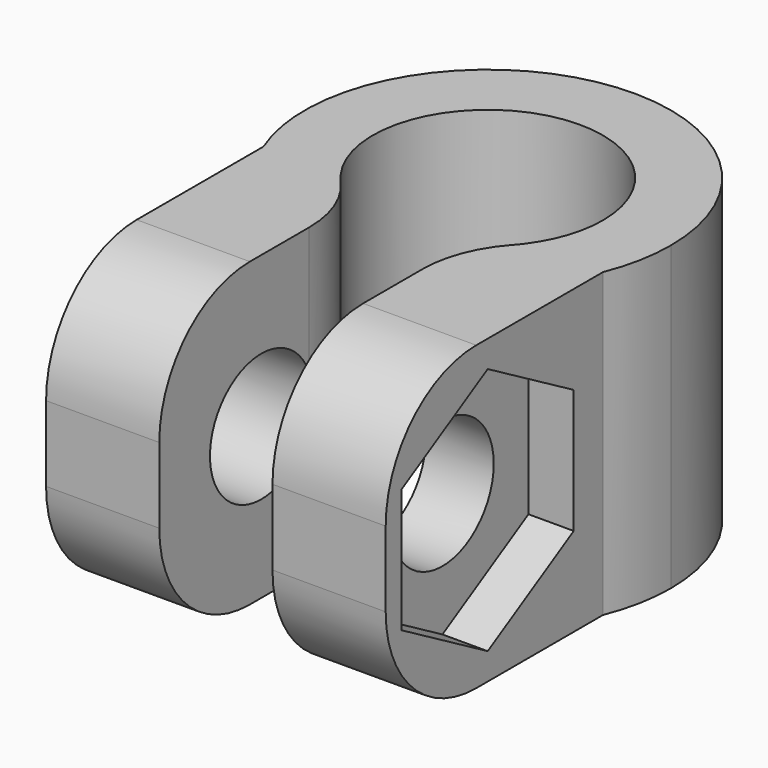
from build123d import *

# Parameters (mm, degrees)
F1_DEPTH    = 8
F2_R        = 1.7
F3_DEPTH    = 9.351
F2_R_2      = 2.75
F4_DEPTH    = 1.2
F5_T1_DEPTH = 14.9408405207
F5_T3_DEPTH = 18
F5_T5_DEPTH = 18


# Not quite as in the source:
# - a fillet or chamfer that OpenCascade refuses, or shapes differently, is made with other operations: its cross-section is extruded or revolved along the edge and cut away or added


with BuildPart() as f1:
    # F0 (on Top) → F1 (new body)
    with BuildSketch(Plane.XY):
        with BuildLine():
            Line((-1.5, -4.6122120506), (-1.5, -2.655654345))
            ThreePointArc((-1.5, -2.655654345), (-2.022599329, -2.2828911394), (-2.4556058316, -1.8090052515))
            Line((-2.4556058316, -1.8090052515), (-4.5, -1.8090052515))
            ThreePointArc((-4.5, -1.8090052515), (-3.3112674446, -3.5437279679), (-1.5, -4.6122120506))
        make_face()
        with BuildLine():
            ThreePointArc((2.4556058316, -1.8090052515), (2.022599329, -2.2828911394), (1.5, -2.655654345))
            Line((1.5, -2.655654345), (1.5, -4.6122120506))
            ThreePointArc((1.5, -4.6122120506), (3.3112674446, -3.5437279679), (4.5, -1.8090052515))
            Line((4.5, -1.8090052515), (2.4556058316, -1.8090052515))
        make_face()
        with BuildLine():
            ThreePointArc((4.5, -1.8090052515), (3.3112674446, -3.5437279679), (1.5, -4.6122120506))
            Line((1.5, -4.6122120506), (1.5, -9.0090052515))
            Line((1.5, -9.0090052515), (4.5, -9.0090052515))
            Line((4.5, -9.0090052515), (4.5, -1.8090052515))
        make_face()
        with BuildLine():
            Line((-1.5, -9.0090052515), (-1.5, -4.6122120506))
            ThreePointArc((-1.5, -4.6122120506), (-3.3112674446, -3.5437279679), (-4.5, -1.8090052515))
            Line((-4.5, -1.8090052515), (-4.5, -9.0090052515))
            Line((-4.5, -9.0090052515), (-1.5, -9.0090052515))
        make_face()
        with BuildLine():
            Line((-4.5, -1.8090052515), (-2.4556058316, -1.8090052515))
            ThreePointArc((-2.4556058316, -1.8090052515), (-0.9520772589, 2.8975936384), (3.05, 0))
            ThreePointArc((3.05, 0), (2.8975936384, -0.9520772589), (2.4556058316, -1.8090052515))
            Line((2.4556058316, -1.8090052515), (4.5, -1.8090052515))
            ThreePointArc((4.5, -1.8090052515), (4.7616961264, -0.9212762886), (4.85, 0))
            ThreePointArc((4.85, 0), (-0.9212762886, 4.7616961264), (-4.5, -1.8090052515))
        make_face()
    extrude(amount=F1_DEPTH)

    # F2 (on face) → F3 (cut, through all)
    with BuildSketch(Plane.YZ.offset(4.5)):
        with Locations((-5.6298957206, 4)):
            Circle(F2_R)
    extrude(amount=-F3_DEPTH, mode=Mode.SUBTRACT)

    # F2 (on face) → F4 (cut)
    with BuildSketch(Plane.YZ.offset(4.5)):
        Polygon((-8.4798957206, 5.6454482672), (-8.4798957206, 2.3545517328), (-5.6298957206, 0.7091034656), (-2.7798957206, 2.3545517328), (-2.7798957206, 5.6454482672), (-5.6298957206, 7.2908965344), align=None)
        with Locations((-5.6298957206, 4)):
            Circle(F2_R_2, mode=Mode.SUBTRACT)
        with Locations((-5.6298957206, 4)):
            Circle(F2_R_2)
        with Locations((-5.6298957206, 4)):
            Circle(F2_R, mode=Mode.SUBTRACT)
    extrude(amount=-F4_DEPTH, mode=Mode.SUBTRACT)

    # F5: fillet of radius 3 on 6 edges, made by hand

    # F5_s2 → F5_t1 (cut)
    with BuildSketch(Plane.XY.offset(-3.4704202604)):
        with BuildLine():
            ThreePointArc((2.2685950413, -2.0386212347), (1.6987311022, -2.9700941027), (1.5, -4.0438224491))
            Line((1.5, -4.0438224491), (1.5, -2.655654345))
            ThreePointArc((1.5, -2.655654345), (1.9093872345, -2.3783902936), (2.2685950413, -2.0386212347))
        make_face()
        with BuildLine():
            ThreePointArc((-1.5, -4.0438224491), (-1.6987311022, -2.9700941027), (-2.2685950413, -2.0386212347))
            ThreePointArc((-2.2685950413, -2.0386212347), (-1.9093872345, -2.3783902936), (-1.5, -2.655654345))
            Line((-1.5, -2.655654345), (-1.5, -4.0438224491))
        make_face()
    extrude(amount=F5_T1_DEPTH, mode=Mode.SUBTRACT)

    # F5_s4 → F5_t3 (cut)
    with BuildSketch(Plane.YZ.offset(-6)):
        with BuildLine():
            ThreePointArc((-6.0090052515, 8), (-8.1303255951, 7.1213203436), (-9.0090052515, 5))
            Line((-9.0090052515, 5), (-9.0090052515, 8))
            Line((-9.0090052515, 8), (-6.0090052515, 8))
        make_face()
        with BuildLine():
            ThreePointArc((-6.0090052515, 0), (-8.1303255951, 0.8786796564), (-9.0090052515, 3))
            Line((-9.0090052515, 3), (-9.0090052515, 0))
            Line((-9.0090052515, 0), (-6.0090052515, 0))
        make_face()
    extrude(amount=F5_T3_DEPTH, mode=Mode.SUBTRACT)

    # F5_s6 → F5_t5 (cut)
    with BuildSketch(Plane.YZ.offset(-12)):
        with BuildLine():
            ThreePointArc((-6.0090052515, 8), (-8.1303255951, 7.1213203436), (-9.0090052515, 5))
            Line((-9.0090052515, 5), (-9.0090052515, 8))
            Line((-9.0090052515, 8), (-6.0090052515, 8))
        make_face()
        with BuildLine():
            ThreePointArc((-6.0090052515, 0), (-8.1303255951, 0.8786796564), (-9.0090052515, 3))
            Line((-9.0090052515, 3), (-9.0090052515, 0))
            Line((-9.0090052515, 0), (-6.0090052515, 0))
        make_face()
    extrude(amount=F5_T5_DEPTH, mode=Mode.SUBTRACT)


solid = f1.part
